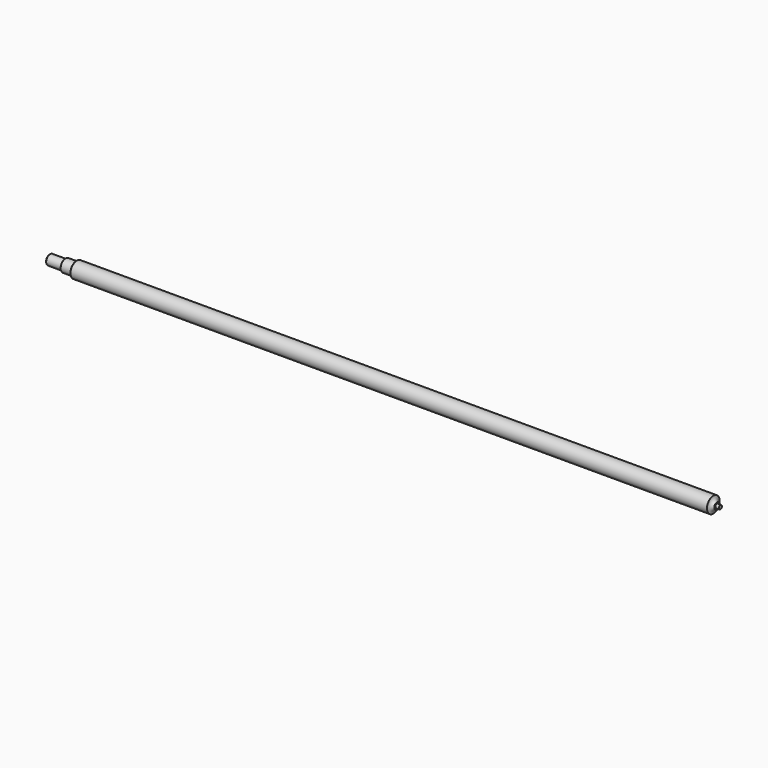
from build123d import *

# Parameters (mm, degrees)
F2_SIZE = 1
F3_SIZE = 0.25
F4_SIZE = 1


with BuildPart() as f1:
    # F0 (on Front) → F1 (revolve)
    with BuildSketch(Plane.XZ):
        with BuildLine():
            Line((-39.6347922059, 59.4147157063), (-39.6347922059, 49.4147157063))
            Line((-39.6347922059, 49.4147157063), (1315.9418255951, 49.4147157063))
            Line((1315.9418255951, 49.4147157063), (1315.9418255951, 53.4147157063))
            Line((1315.9418255951, 53.4147157063), (1308.9418255951, 53.4147157063))
            Line((1308.9418255951, 53.4147157063), (1308.9418255951, 55.9769750426))
            ThreePointArc((1308.9418255951, 55.9769750426), (1303.814166428, 59.5216123442), (1301.782252331, 65.4147157063))
            Line((1301.782252331, 65.4147157063), (14.3652077941, 65.4147157063))
            Line((14.3652077941, 65.4147157063), (14.3652077941, 61.9147157063))
            Line((14.3652077941, 61.9147157063), (-7.6347922059, 61.9147157063))
            Line((-7.6347922059, 61.9147157063), (-7.6347922059, 59.4147157063))
            Line((-7.6347922059, 59.4147157063), (-39.6347922059, 59.4147157063))
        make_face()
    revolve(axis=Axis((638.1535166946, 0, 49.4147157063), (1, 0, 0)))

    # F2
    f2_edges = [f1.edges().sort_by_distance(p)[0] for p in [
        (14.365208, 0, 33.414716),
    ]]
    chamfer(f2_edges, length=F2_SIZE)

    # F3
    f3_edges = [f1.edges().sort_by_distance(p)[0] for p in [
        (-7.634792, 0, 36.914716),
    ]]
    chamfer(f3_edges, length=F3_SIZE)

    # F4
    f4_edges = [f1.edges().sort_by_distance(p)[0] for p in [
        (-39.634792, 0, 39.414716),
    ]]
    chamfer(f4_edges, length=F4_SIZE)


solid = f1.part
